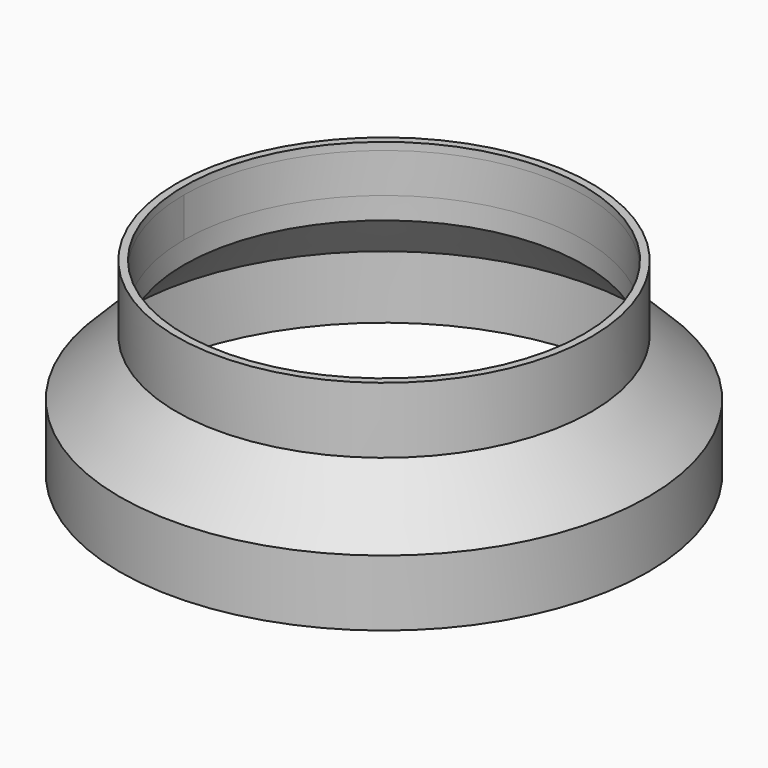
from build123d import *
from build123d import SkipClean  # not in build123d's __all__

# Parameters (mm, degrees)
F2_T     = -4
F3_R     = 106
F4_DEPTH = 25


with BuildPart() as f1:
    # F0 (on Front) → F1 (revolve)
    with BuildSketch(Plane.XZ):
        Polygon((-140, 35), (-140, 0), (0, 0), (0, 100), (-110, 100), (-110, 65), align=None)
    revolve(axis=Axis((0, 0, 50), (0, 0, 1)))

    # F2
    f2_openings = [f1.faces().sort_by_distance(p)[0] for p in [
        (0, 0, 0),
    ]]
    offset(amount=F2_T, openings=f2_openings, kind=Kind.INTERSECTION)

    # F3 (on face) → F4 (cut)
    with BuildSketch(Plane.XY.offset(100)):
        Circle(F3_R)
    with SkipClean():  # cleaning this boolean's faces spoils the solid; the shape is the same uncleaned
        extrude(amount=-F4_DEPTH, mode=Mode.SUBTRACT)


solid = f1.part
